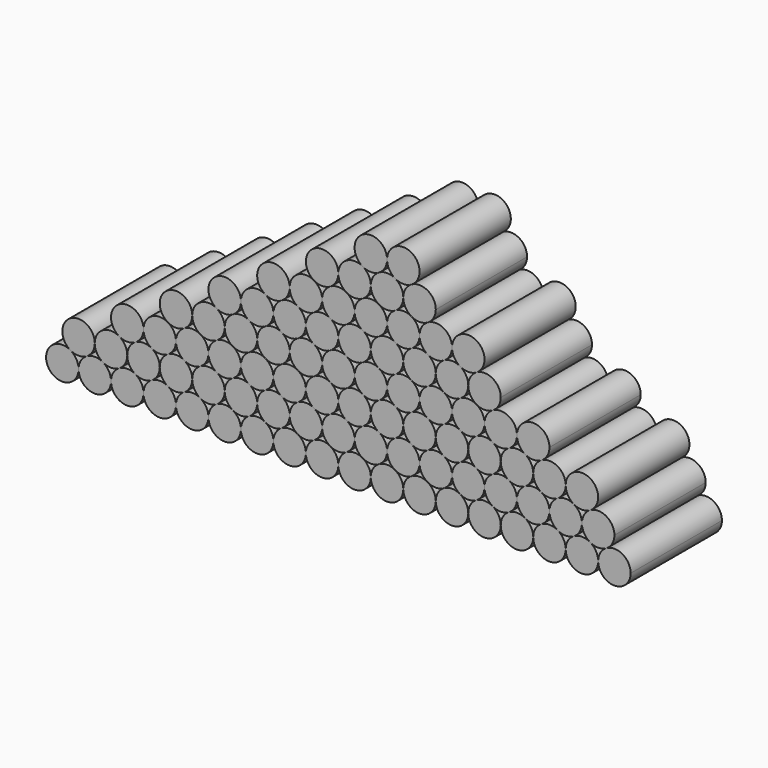
from build123d import *

# Parameters (mm, degrees)
F1_DEPTH = 65


with BuildPart() as f1:
    # F0 (on Front) → F1 (new body)
    with BuildSketch(Plane.XZ):
        with BuildLine():
            ThreePointArc((94.3613596421, 104.9688568004), (90.9756243137, 101.583121778), (89.7363591594, 96.9581215367))
            ThreePointArc((89.7363591594, 96.9581215367), (98.9863591594, 87.7081215367), (108.2363591594, 96.9581215367))
            ThreePointArc((108.2363591594, 96.9581215367), (103.6113594008, 104.9688563823), (94.3613596421, 104.9688568004))
        make_face()
        with BuildLine():
            ThreePointArc((48.1113591587, 137.0117964621), (52.7363591594, 135.7725314467), (57.3613591601, 137.0117964621))
            ThreePointArc((57.3613591601, 137.0117964621), (60.7470941446, 140.397531447), (61.9863591594, 145.0225314467))
            ThreePointArc((61.9863591594, 145.0225314467), (52.7363591594, 154.2725314467), (43.4863591594, 145.0225314467))
            ThreePointArc((43.4863591594, 145.0225314467), (44.7256241742, 140.397531447), (48.1113591587, 137.0117964621))
        make_face()
        with BuildLine():
            ThreePointArc((-25.8886414057, 201.097676668), (-21.2636411008, 199.8584113267), (-16.6386407261, 201.0976764078))
            ThreePointArc((-16.6386407261, 201.0976764078), (-13.2529058226, 204.483411384), (-12.0136408406, 209.1084113267))
            ThreePointArc((-12.0136408406, 209.1084113267), (-21.2636408406, 218.3584113267), (-30.5136408406, 209.1084113267))
            ThreePointArc((-30.5136408406, 209.1084113267), (-29.2743759887, 204.4834116093), (-25.8886414057, 201.097676668))
        make_face()
        with BuildLine():
            ThreePointArc((11.1113595071, 169.054736201), (15.7363595326, 167.8154713867), (20.361359458, 169.0547365741))
            ThreePointArc((20.361359458, 169.0547365741), (23.7470942306, 172.440471536), (24.9863591594, 177.0654713867))
            ThreePointArc((24.9863591594, 177.0654713867), (15.7363591594, 186.3154713867), (6.4863591594, 177.0654713867))
            ThreePointArc((6.4863591594, 177.0654713867), (7.7256242748, 172.4404712129), (11.1113595071, 169.054736201))
        make_face()
        with BuildLine():
            ThreePointArc((-197.0136408406, 112.9795915067), (-210.8886408403, 120.9903264919), (-210.8886408413, 104.9688565221))
            ThreePointArc((-210.8886408413, 104.9688565221), (-206.2636409659, 103.7295915067), (-201.6386410569, 104.9688563968))
            ThreePointArc((-201.6386410569, 104.9688563968), (-198.252905918, 108.3545913985), (-197.0136408406, 112.9795915067))
        make_face()
        with BuildLine():
            ThreePointArc((-183.1386408399, 120.9903264913), (-178.5136408406, 119.7510614767), (-173.8886408413, 120.9903264913))
            ThreePointArc((-173.8886408413, 120.9903264913), (-170.5029058558, 124.3760614763), (-169.2636408406, 129.0010614767))
            ThreePointArc((-169.2636408406, 129.0010614767), (-183.138640841, 137.0117964615), (-183.1386408399, 120.9903264913))
        make_face()
        with BuildLine():
            ThreePointArc((-155.3886408399, 137.0117964613), (-150.7636408406, 135.7725314467), (-146.1386408413, 137.0117964613))
            ThreePointArc((-146.1386408413, 137.0117964613), (-142.7529058558, 140.3975314464), (-141.5136408406, 145.0225314467))
            ThreePointArc((-141.5136408406, 145.0225314467), (-155.388640841, 153.0332664315), (-155.3886408399, 137.0117964613))
        make_face()
        with BuildLine():
            ThreePointArc((-127.6386408399, 153.0332664313), (-123.0136408406, 151.7940014167), (-118.3886408413, 153.0332664313))
            ThreePointArc((-118.3886408413, 153.0332664313), (-115.0029058558, 156.4190014164), (-113.7636408406, 161.0440014167))
            ThreePointArc((-113.7636408406, 161.0440014167), (-127.638640841, 169.0547364015), (-127.6386408399, 153.0332664313))
        make_face()
        with BuildLine():
            ThreePointArc((-86.0136408406, 177.0654713867), (-99.888640841, 185.0762063715), (-99.8886408399, 169.0547364013))
            ThreePointArc((-99.8886408399, 169.0547364013), (-95.2636408406, 167.8154713867), (-90.6386408413, 169.0547364013))
            ThreePointArc((-90.6386408413, 169.0547364013), (-87.2529058558, 172.4404713864), (-86.0136408406, 177.0654713867))
        make_face()
        with BuildLine():
            ThreePointArc((-58.2636408406, 193.0869413567), (-72.1386405587, 201.0976765045), (-72.1386414043, 185.0762066972))
            ThreePointArc((-72.1386414043, 185.0762066972), (-67.5136407818, 183.8369413567), (-62.8886401751, 185.076206756))
            ThreePointArc((-62.8886401751, 185.076206756), (-59.5029056635, 188.4619416895), (-58.2636408406, 193.0869413567))
        make_face()
        with BuildLine():
            ThreePointArc((-44.3886404911, 201.0976761399), (-39.7636403903, 199.8584113267), (-35.1386404101, 201.0976765903))
            ThreePointArc((-35.1386404101, 201.0976765903), (-31.7529057313, 204.483411542), (-30.5136408406, 209.1084113267))
            ThreePointArc((-30.5136408406, 209.1084113267), (-44.3886410154, 217.1191462109), (-44.3886404911, 201.0976761399))
        make_face()
        with BuildLine():
            ThreePointArc((75.8613592919, 120.9903264151), (80.4863592363, 119.7510614767), (85.1113591601, 120.9903264921))
            ThreePointArc((85.1113591601, 120.9903264921), (88.4970941446, 124.376061477), (89.7363591594, 129.0010614767))
            ThreePointArc((89.7363591594, 129.0010614767), (80.4863591594, 138.2510614767), (71.2363591594, 129.0010614767))
            ThreePointArc((71.2363591594, 129.0010614767), (72.4756242127, 124.3760614104), (75.8613592919, 120.9903264151))
        make_face()
        with BuildLine():
            ThreePointArc((71.2363591594, 96.9581215367), (80.4863591594, 87.7081215367), (89.7363591594, 96.9581215367))
            ThreePointArc((89.7363591594, 96.9581215367), (88.4970943958, 101.5831211012), (85.1113600303, 104.9688560188))
            ThreePointArc((85.1113600303, 104.9688560188), (80.4863599409, 106.2081215367), (75.8613596421, 104.9688568004))
            ThreePointArc((75.8613596421, 104.9688568004), (72.4756243137, 101.583121778), (71.2363591594, 96.9581215367))
        make_face()
        with BuildLine():
            ThreePointArc((34.2363591594, 96.9581215367), (43.4863591594, 87.7081215367), (52.7363591594, 96.9581215367))
            ThreePointArc((52.7363591594, 96.9581215367), (51.4970944116, 101.5831210738), (48.1113600851, 104.9688559872))
            ThreePointArc((48.1113600851, 104.9688559872), (43.4863593684, 106.2081215367), (38.8613585957, 104.9688561962))
            ThreePointArc((38.8613585957, 104.9688561962), (35.4756240116, 101.5831212548), (34.2363591594, 96.9581215367))
        make_face()
        with BuildLine():
            ThreePointArc((15.7363591594, 96.9581215367), (24.9863591594, 87.7081215367), (34.2363591594, 96.9581215367))
            ThreePointArc((34.2363591594, 96.9581215367), (32.9970943988, 101.5831210961), (29.6113600405, 104.968856013))
            ThreePointArc((29.6113600405, 104.968856013), (24.9863592931, 106.2081215367), (20.3613585098, 104.9688561466))
            ThreePointArc((20.3613585098, 104.9688561466), (16.9756239869, 101.5831212119), (15.7363591594, 96.9581215367))
        make_face()
        with BuildLine():
            ThreePointArc((52.7363591594, 96.9581215367), (61.9863591594, 87.7081215367), (71.2363591594, 96.9581215367))
            ThreePointArc((71.2363591594, 96.9581215367), (69.9970944022, 101.5831210901), (66.6113600525, 104.968856006))
            ThreePointArc((66.6113600525, 104.968856006), (61.9863592726, 106.2081215367), (57.3613584624, 104.9688561193))
            ThreePointArc((57.3613584624, 104.9688561193), (53.9756239732, 101.5831211882), (52.7363591594, 96.9581215367))
        make_face()
        with BuildLine():
            ThreePointArc((-113.7636408406, 96.9581215367), (-104.5136408406, 87.7081215367), (-95.2636408406, 96.9581215367))
            ThreePointArc((-95.2636408406, 96.9581215367), (-96.5029058558, 101.583121537), (-99.8886408413, 104.9688565221))
            ThreePointArc((-99.8886408413, 104.9688565221), (-104.5136408406, 106.2081215367), (-109.1386408399, 104.9688565221))
            ThreePointArc((-109.1386408399, 104.9688565221), (-112.5243758254, 101.583121537), (-113.7636408406, 96.9581215367))
        make_face()
        with BuildLine():
            ThreePointArc((-95.2636408406, 96.9581215367), (-86.0136408406, 87.7081215367), (-76.7636408406, 96.9581215367))
            ThreePointArc((-76.7636408406, 96.9581215367), (-78.0029058528, 101.5831215319), (-81.388640831, 104.9688565161))
            ThreePointArc((-81.388640831, 104.9688565161), (-86.0136405564, 106.2081215367), (-90.6386403578, 104.9688568004))
            ThreePointArc((-90.6386403578, 104.9688568004), (-94.0243756863, 101.583121778), (-95.2636408406, 96.9581215367))
        make_face()
        with BuildLine():
            ThreePointArc((-76.7636408406, 96.9581215367), (-67.5136408406, 87.7081215367), (-58.2636408406, 96.9581215367))
            ThreePointArc((-58.2636408406, 96.9581215367), (-59.5029057551, 101.5831213626), (-62.8886404925, 104.9688563207))
            ThreePointArc((-62.8886404925, 104.9688563207), (-67.5136406392, 106.2081215367), (-72.1386408399, 104.9688565221))
            ThreePointArc((-72.1386408399, 104.9688565221), (-75.5243758254, 101.583121537), (-76.7636408406, 96.9581215367))
        make_face()
        with BuildLine():
            ThreePointArc((-58.2636408406, 96.9581215367), (-49.0136408406, 87.7081215367), (-39.7636408406, 96.9581215367))
            ThreePointArc((-39.7636408406, 96.9581215367), (-41.0029057637, 101.5831213774), (-44.3886405222, 104.9688563378))
            ThreePointArc((-44.3886405222, 104.9688563378), (-49.0136408578, 106.2081215367), (-53.6386411888, 104.9688563207))
            ThreePointArc((-53.6386411888, 104.9688563207), (-57.0243759261, 101.5831213626), (-58.2636408406, 96.9581215367))
        make_face()
        with BuildLine():
            ThreePointArc((-39.7636408406, 96.9581215367), (-30.5136408406, 87.7081215367), (-21.2636408406, 96.9581215367))
            ThreePointArc((-21.2636408406, 96.9581215367), (-22.5029057222, 101.5831213057), (-25.8886403787, 104.968856255))
            ThreePointArc((-25.8886403787, 104.968856255), (-30.5136403721, 106.2081215367), (-35.1386404911, 104.9688567235))
            ThreePointArc((-35.1386404911, 104.9688567235), (-38.5243757247, 101.5831217114), (-39.7636408406, 96.9581215367))
        make_face()
        with BuildLine():
            ThreePointArc((-21.2636408406, 96.9581215367), (-12.0136408406, 87.7081215367), (-2.7636408406, 96.9581215367))
            ThreePointArc((-2.7636408406, 96.9581215367), (-4.0029056931, 101.5831212551), (-7.3886402775, 104.9688561966))
            ThreePointArc((-7.3886402775, 104.9688561966), (-12.0136406984, 106.2081215367), (-16.6386411573, 104.9688563388))
            ThreePointArc((-16.6386411573, 104.9688563388), (-20.024375917, 101.5831213783), (-21.2636408406, 96.9581215367))
        make_face()
        with BuildLine():
            ThreePointArc((85.1113600303, 104.9688560188), (89.7363599409, 103.7295915067), (94.3613596421, 104.9688568004))
            ThreePointArc((94.3613596421, 104.9688568004), (97.7470942838, 108.3545917481), (98.9863591594, 112.9795915067))
            ThreePointArc((98.9863591594, 112.9795915067), (94.3613591597, 120.9903264915), (85.1113591601, 120.9903264921))
            ThreePointArc((85.1113591601, 120.9903264921), (81.7256241746, 117.604591507), (80.4863591594, 112.9795915067))
            ThreePointArc((80.4863591594, 112.9795915067), (81.7256244258, 108.3545910712), (85.1113600303, 104.9688560188))
        make_face()
        with BuildLine():
            ThreePointArc((-2.7636408406, 96.9581215367), (6.4863591594, 87.7081215367), (15.7363591594, 96.9581215367))
            ThreePointArc((15.7363591594, 96.9581215367), (14.4970942484, 101.5831213566), (11.1113595196, 104.9688563137))
            ThreePointArc((11.1113595196, 104.9688563137), (6.4863591482, 106.2081215367), (1.8613587798, 104.9688563025))
            ThreePointArc((1.8613587798, 104.9688563025), (-1.5243759352, 101.5831213469), (-2.7636408406, 96.9581215367))
        make_face()
        with BuildLine():
            ThreePointArc((-206.2636408406, 96.9581215367), (-197.0136408406, 87.7081215367), (-187.7636408406, 96.9581215367))
            ThreePointArc((-187.7636408406, 96.9581215367), (-189.0029057551, 101.5831213626), (-192.3886404925, 104.9688563207))
            ThreePointArc((-192.3886404925, 104.9688563207), (-197.0136407645, 106.2081215367), (-201.6386410569, 104.9688563968))
            ThreePointArc((-201.6386410569, 104.9688563968), (-205.024375888, 101.5831214285), (-206.2636408406, 96.9581215367))
        make_face()
        with BuildLine():
            ThreePointArc((-187.7636408406, 96.9581215367), (-178.5136408406, 87.7081215367), (-169.2636408406, 96.9581215367))
            ThreePointArc((-169.2636408406, 96.9581215367), (-170.5029058554, 101.5831215363), (-173.8886408399, 104.9688565213))
            ThreePointArc((-173.8886408399, 104.9688565213), (-178.5136408398, 106.2081215367), (-183.1386408399, 104.9688565221))
            ThreePointArc((-183.1386408399, 104.9688565221), (-186.5243758254, 101.583121537), (-187.7636408406, 96.9581215367))
        make_face()
        with BuildLine():
            ThreePointArc((-169.2636408406, 96.9581215367), (-160.0136408406, 87.7081215367), (-150.7636408406, 96.9581215367))
            ThreePointArc((-150.7636408406, 96.9581215367), (-152.0029058472, 101.5831215222), (-155.3886408116, 104.9688565049))
            ThreePointArc((-155.3886408116, 104.9688565049), (-160.0136406229, 106.2081215367), (-164.6386404925, 104.9688567227))
            ThreePointArc((-164.6386404925, 104.9688567227), (-168.0243757251, 101.5831217107), (-169.2636408406, 96.9581215367))
        make_face()
        with BuildLine():
            ThreePointArc((-150.7636408406, 96.9581215367), (-141.5136408406, 87.7081215367), (-132.2636408406, 96.9581215367))
            ThreePointArc((-132.2636408406, 96.9581215367), (-133.5029057936, 101.5831214292), (-136.8886406257, 104.9688563976))
            ThreePointArc((-136.8886406257, 104.9688563976), (-141.5136407161, 106.2081215367), (-146.1386408399, 104.9688565221))
            ThreePointArc((-146.1386408399, 104.9688565221), (-149.5243758254, 101.583121537), (-150.7636408406, 96.9581215367))
        make_face()
        with BuildLine():
            ThreePointArc((-132.2636408406, 96.9581215367), (-123.0136408406, 87.7081215367), (-113.7636408406, 96.9581215367))
            ThreePointArc((-113.7636408406, 96.9581215367), (-115.0029058558, 101.583121537), (-118.3886408413, 104.9688565221))
            ThreePointArc((-118.3886408413, 104.9688565221), (-123.0136405576, 106.2081215367), (-127.6386403497, 104.9688568051))
            ThreePointArc((-127.6386403497, 104.9688568051), (-131.0243756839, 101.5831217821), (-132.2636408406, 96.9581215367))
        make_face()
        with BuildLine():
            ThreePointArc((20.3613591587, 153.0332664321), (24.9863592839, 151.7940014167), (29.6113593757, 153.0332665566))
            ThreePointArc((29.6113593757, 153.0332665566), (32.9970942068, 156.4190015248), (34.2363591594, 161.0440014167))
            ThreePointArc((34.2363591594, 161.0440014167), (29.6113593087, 169.0547363155), (20.361359458, 169.0547365741))
            ThreePointArc((20.361359458, 169.0547365741), (16.9756242606, 165.669001566), (15.7363591594, 161.0440014167))
            ThreePointArc((15.7363591594, 161.0440014167), (16.9756241742, 156.4190014171), (20.3613591587, 153.0332664321))
        make_face()
        with BuildLine():
            ThreePointArc((-16.6386408413, 185.0762063721), (-12.0136407594, 183.8369413567), (-7.3886406993, 185.0762064533))
            ThreePointArc((-7.3886406993, 185.0762064533), (-4.0029058148, 188.4619414274), (-2.7636408406, 193.0869413567))
            ThreePointArc((-2.7636408406, 193.0869413567), (-7.3886407834, 201.0976763087), (-16.6386407261, 201.0976764078))
            ThreePointArc((-16.6386407261, 201.0976764078), (-20.0243757926, 197.711941414), (-21.2636408406, 193.0869413567))
            ThreePointArc((-21.2636408406, 193.0869413567), (-20.0243758258, 188.4619413571), (-16.6386408413, 185.0762063721))
        make_face()
        with BuildLine():
            ThreePointArc((-197.0136408406, 112.9795915067), (-195.7743757251, 108.3545913326), (-192.3886404925, 104.9688563207))
            ThreePointArc((-192.3886404925, 104.9688563207), (-187.7636406392, 103.7295915067), (-183.1386408399, 104.9688565221))
            ThreePointArc((-183.1386408399, 104.9688565221), (-179.7529058554, 108.354591507), (-178.5136408406, 112.9795915067))
            ThreePointArc((-178.5136408406, 112.9795915067), (-179.7529058554, 117.6045915063), (-183.1386408399, 120.9903264913))
            ThreePointArc((-183.1386408399, 120.9903264913), (-192.3886408403, 120.9903264919), (-197.0136408406, 112.9795915067))
        make_face()
        with BuildLine():
            ThreePointArc((-169.2636408406, 129.0010614767), (-168.0243757636, 124.3760613692), (-164.6386406257, 120.9903263676))
            ThreePointArc((-164.6386406257, 120.9903263676), (-160.0136407161, 119.7510614767), (-155.3886408399, 120.9903264921))
            ThreePointArc((-155.3886408399, 120.9903264921), (-152.0029058554, 124.376061477), (-150.7636408406, 129.0010614767))
            ThreePointArc((-150.7636408406, 129.0010614767), (-152.0029058554, 133.6260614763), (-155.3886408399, 137.0117964613))
            ThreePointArc((-155.3886408399, 137.0117964613), (-164.6386408403, 137.0117964619), (-169.2636408406, 129.0010614767))
        make_face()
        with BuildLine():
            ThreePointArc((57.3613591273, 120.9903265102), (61.9863591888, 119.7510614767), (66.6113592424, 120.9903265396))
            ThreePointArc((66.6113592424, 120.9903265396), (69.9970941684, 124.3760615182), (71.2363591594, 129.0010614767))
            ThreePointArc((71.2363591594, 129.0010614767), (66.6113591597, 137.0117964615), (57.3613591601, 137.0117964621))
            ThreePointArc((57.3613591601, 137.0117964621), (53.9756241746, 133.626061477), (52.7363591594, 129.0010614767))
            ThreePointArc((52.7363591594, 129.0010614767), (53.9756241651, 124.3760614928), (57.3613591273, 120.9903265102))
        make_face()
        with BuildLine():
            ThreePointArc((-141.5136408406, 145.0225314467), (-140.2743757251, 140.3975312726), (-136.8886404925, 137.0117962607))
            ThreePointArc((-136.8886404925, 137.0117962607), (-132.2636406392, 135.7725314467), (-127.6386408399, 137.0117964621))
            ThreePointArc((-127.6386408399, 137.0117964621), (-124.2529058554, 140.397531447), (-123.0136408406, 145.0225314467))
            ThreePointArc((-123.0136408406, 145.0225314467), (-124.2529058554, 149.6475314464), (-127.6386408399, 153.0332664313))
            ThreePointArc((-127.6386408399, 153.0332664313), (-136.8886408403, 153.0332664319), (-141.5136408406, 145.0225314467))
        make_face()
        with BuildLine():
            ThreePointArc((-109.138640708, 153.0332663552), (-104.5136407637, 151.7940014167), (-99.8886408399, 153.0332664321))
            ThreePointArc((-99.8886408399, 153.0332664321), (-96.5029058554, 156.4190014171), (-95.2636408406, 161.0440014167))
            ThreePointArc((-95.2636408406, 161.0440014167), (-96.5029058554, 165.6690014164), (-99.8886408399, 169.0547364013))
            ThreePointArc((-99.8886408399, 169.0547364013), (-109.1386408403, 169.0547364019), (-113.7636408406, 161.0440014167))
            ThreePointArc((-113.7636408406, 161.0440014167), (-112.5243757873, 156.4190013504), (-109.138640708, 153.0332663552))
        make_face()
        with BuildLine():
            ThreePointArc((29.6113595134, 137.0117962573), (34.2363593679, 135.7725314467), (38.8613591664, 137.0117964657))
            ThreePointArc((38.8613591664, 137.0117964657), (42.2470941464, 140.3975314502), (43.4863591594, 145.0225314467))
            ThreePointArc((43.4863591594, 145.0225314467), (38.8613592675, 153.0332663693), (29.6113593757, 153.0332665566))
            ThreePointArc((29.6113593757, 153.0332665566), (26.2256242368, 149.6475315548), (24.9863591594, 145.0225314467))
            ThreePointArc((24.9863591594, 145.0225314467), (26.2256242766, 140.3975312697), (29.6113595134, 137.0117962573))
        make_face()
        with BuildLine():
            ThreePointArc((-86.0136408406, 177.0654713867), (-84.7743757873, 172.4404713203), (-81.3886407078, 169.0547363251))
            ThreePointArc((-81.3886407078, 169.0547363251), (-76.7636407636, 167.8154713867), (-72.1386408399, 169.0547364021))
            ThreePointArc((-72.1386408399, 169.0547364021), (-68.7529058554, 172.4404713871), (-67.5136408406, 177.0654713867))
            ThreePointArc((-67.5136408406, 177.0654713867), (-68.7529060183, 181.6904716686), (-72.1386414043, 185.0762066972))
            ThreePointArc((-72.1386414043, 185.0762066972), (-81.3886411225, 185.076206209), (-86.0136408406, 177.0654713867))
        make_face()
        with BuildLine():
            ThreePointArc((-12.0136408406, 177.0654713867), (-10.7743759018, 172.4404715188), (-7.3886411047, 169.0547365542))
            ThreePointArc((-7.3886411047, 169.0547365542), (-2.7636411967, 167.8154713867), (1.8613588067, 169.0547361981))
            ThreePointArc((1.8613588067, 169.0547361981), (5.2470940426, 172.4404712104), (6.4863591594, 177.0654713867))
            ThreePointArc((6.4863591594, 177.0654713867), (1.8613592301, 185.0762063309), (-7.3886406993, 185.0762064533))
            ThreePointArc((-7.3886406993, 185.0762064533), (-10.7743757848, 181.6904714574), (-12.0136408406, 177.0654713867))
        make_face()
        with BuildLine():
            ThreePointArc((-53.6386408155, 185.0762063572), (-49.0136407012, 183.8369413567), (-44.3886406243, 185.0762064966))
            ThreePointArc((-44.3886406243, 185.0762064966), (-41.0029057932, 188.4619414649), (-39.7636408406, 193.0869413567))
            ThreePointArc((-39.7636408406, 193.0869413567), (-41.0029057547, 197.711941182), (-44.3886404911, 201.0976761399))
            ThreePointArc((-44.3886404911, 201.0976761399), (-53.6386406659, 201.0976764426), (-58.2636408406, 193.0869413567))
            ThreePointArc((-58.2636408406, 193.0869413567), (-57.0243758184, 188.4619413442), (-53.6386408155, 185.0762063572))
        make_face()
        with BuildLine():
            ThreePointArc((-86.0136408406, 145.0225314467), (-84.7743758258, 140.397531447), (-81.3886408413, 137.0117964621))
            ThreePointArc((-81.3886408413, 137.0117964621), (-76.7636408406, 135.7725314467), (-72.1386408399, 137.0117964621))
            ThreePointArc((-72.1386408399, 137.0117964621), (-68.7529058554, 140.397531447), (-67.5136408406, 145.0225314467))
            ThreePointArc((-67.5136408406, 145.0225314467), (-68.7529058558, 149.647531447), (-72.1386408413, 153.0332664321))
            ThreePointArc((-72.1386408413, 153.0332664321), (-76.7636407161, 154.2725314467), (-81.3886406243, 153.0332665566))
            ThreePointArc((-81.3886406243, 153.0332665566), (-84.7743757632, 149.6475315548), (-86.0136408406, 145.0225314467))
        make_face()
        with BuildLine():
            ThreePointArc((15.7363591594, 129.0010614767), (16.9756241742, 124.376061477), (20.3613591587, 120.9903264921))
            ThreePointArc((20.3613591587, 120.9903264921), (24.9863592069, 119.7510614767), (29.6113592424, 120.9903265396))
            ThreePointArc((29.6113592424, 120.9903265396), (32.9970941684, 124.3760615182), (34.2363591594, 129.0010614767))
            ThreePointArc((34.2363591594, 129.0010614767), (32.9970942466, 133.6260612997), (29.6113595134, 137.0117962573))
            ThreePointArc((29.6113595134, 137.0117962573), (24.9863592389, 138.2510614767), (20.3613589431, 137.0117963368))
            ThreePointArc((20.3613589431, 137.0117963368), (16.975624112, 133.6260613685), (15.7363591594, 129.0010614767))
        make_face()
        with BuildLine():
            ThreePointArc((29.6113600405, 104.968856013), (34.2363593426, 103.7295915067), (38.8613585957, 104.9688561962))
            ThreePointArc((38.8613585957, 104.9688561962), (42.2470939817, 108.3545912248), (43.4863591594, 112.9795915067))
            ThreePointArc((43.4863591594, 112.9795915067), (42.2470941827, 117.6045914404), (38.8613592919, 120.9903264151))
            ThreePointArc((38.8613592919, 120.9903264151), (34.2363592839, 122.2295915067), (29.6113592424, 120.9903265396))
            ThreePointArc((29.6113592424, 120.9903265396), (26.2256241984, 117.6045915482), (24.9863591594, 112.9795915067))
            ThreePointArc((24.9863591594, 112.9795915067), (26.2256244287, 108.3545910661), (29.6113600405, 104.968856013))
        make_face()
        with BuildLine():
            ThreePointArc((-12.0136408406, 112.9795915067), (-10.7743756631, 108.3545912251), (-7.3886402775, 104.9688561966))
            ThreePointArc((-7.3886402775, 104.9688561966), (-2.7636407347, 103.7295915067), (1.8613587798, 104.9688563025))
            ThreePointArc((1.8613587798, 104.9688563025), (5.2470940348, 108.3545913169), (6.4863591594, 112.9795915067))
            ThreePointArc((6.4863591594, 112.9795915067), (5.2470941451, 117.6045915055), (1.8613591618, 120.9903264903))
            ThreePointArc((1.8613591618, 120.9903264903), (-2.7636408396, 122.2295915067), (-7.3886408413, 120.9903264913))
            ThreePointArc((-7.3886408413, 120.9903264913), (-10.7743758258, 117.6045915063), (-12.0136408406, 112.9795915067))
        make_face()
        with BuildLine():
            ThreePointArc((-21.2636408406, 129.0010614767), (-20.0243758254, 124.3760614763), (-16.6386408399, 120.9903264913))
            ThreePointArc((-16.6386408399, 120.9903264913), (-12.0136408406, 119.7510614767), (-7.3886408413, 120.9903264913))
            ThreePointArc((-7.3886408413, 120.9903264913), (-4.0029058558, 124.3760614763), (-2.7636408406, 129.0010614767))
            ThreePointArc((-2.7636408406, 129.0010614767), (-4.0029057941, 133.6260613701), (-7.3886406275, 137.0117963386))
            ThreePointArc((-7.3886406275, 137.0117963386), (-12.0136407171, 138.2510614767), (-16.6386408399, 137.0117964621))
            ThreePointArc((-16.6386408399, 137.0117964621), (-20.0243758254, 133.626061477), (-21.2636408406, 129.0010614767))
        make_face()
        with BuildLine():
            ThreePointArc((43.4863591594, 112.9795915067), (44.7256244416, 108.3545910438), (48.1113600851, 104.9688559872))
            ThreePointArc((48.1113600851, 104.9688559872), (52.7363592914, 103.7295915067), (57.3613584624, 104.9688561193))
            ThreePointArc((57.3613584624, 104.9688561193), (60.7470939432, 108.3545911582), (61.9863591594, 112.9795915067))
            ThreePointArc((61.9863591594, 112.9795915067), (60.7470941351, 117.6045915227), (57.3613591273, 120.9903265102))
            ThreePointArc((57.3613591273, 120.9903265102), (52.7363591412, 122.2295915067), (48.1113591601, 120.9903264921))
            ThreePointArc((48.1113591601, 120.9903264921), (44.7256241746, 117.604591507), (43.4863591594, 112.9795915067))
        make_face()
        with BuildLine():
            ThreePointArc((-7.3886406275, 137.0117963386), (-2.7636406402, 135.7725314467), (1.8613592934, 137.0117965391))
            ThreePointArc((1.8613592934, 137.0117965391), (5.2470941831, 140.3975315137), (6.4863591594, 145.0225314467))
            ThreePointArc((6.4863591594, 145.0225314467), (5.2470941442, 149.647531447), (1.8613591587, 153.0332664321))
            ThreePointArc((1.8613591587, 153.0332664321), (-2.7636407594, 154.2725314467), (-7.3886406993, 153.0332665133))
            ThreePointArc((-7.3886406993, 153.0332665133), (-10.7743757848, 149.6475315174), (-12.0136408406, 145.0225314467))
            ThreePointArc((-12.0136408406, 145.0225314467), (-10.7743757641, 140.3975313401), (-7.3886406275, 137.0117963386))
        make_face()
        with BuildLine():
            ThreePointArc((-49.0136408406, 177.0654713867), (-47.7743758184, 172.4404713742), (-44.3886408155, 169.0547363872))
            ThreePointArc((-44.3886408155, 169.0547363872), (-39.7636407488, 167.8154713867), (-35.1386407067, 169.054736479))
            ThreePointArc((-35.1386407067, 169.054736479), (-31.7529058169, 172.4404714537), (-30.5136408406, 177.0654713867))
            ThreePointArc((-30.5136408406, 177.0654713867), (-31.752905918, 181.6904714949), (-35.1386410569, 185.0762064966))
            ThreePointArc((-35.1386410569, 185.0762064966), (-39.7636408406, 186.3154713867), (-44.3886406243, 185.0762064966))
            ThreePointArc((-44.3886406243, 185.0762064966), (-47.7743757632, 181.6904714949), (-49.0136408406, 177.0654713867))
        make_face()
        with BuildLine():
            ThreePointArc((-132.2636408406, 129.0010614767), (-131.0243758258, 124.376061477), (-127.6386408413, 120.9903264921))
            ThreePointArc((-127.6386408413, 120.9903264921), (-123.0136408406, 119.7510614767), (-118.3886408399, 120.9903264921))
            ThreePointArc((-118.3886408399, 120.9903264921), (-115.0029058554, 124.376061477), (-113.7636408406, 129.0010614767))
            ThreePointArc((-113.7636408406, 129.0010614767), (-115.0029057936, 133.6260613692), (-118.3886406257, 137.0117963376))
            ThreePointArc((-118.3886406257, 137.0117963376), (-123.0136407161, 138.2510614767), (-127.6386408399, 137.0117964621))
            ThreePointArc((-127.6386408399, 137.0117964621), (-131.0243758254, 133.626061477), (-132.2636408406, 129.0010614767))
        make_face()
        with BuildLine():
            ThreePointArc((-21.2636408406, 161.0440014167), (-20.0243758258, 156.4190014171), (-16.6386408413, 153.0332664321))
            ThreePointArc((-16.6386408413, 153.0332664321), (-12.0136407594, 151.7940014167), (-7.3886406993, 153.0332665133))
            ThreePointArc((-7.3886406993, 153.0332665133), (-4.0029058148, 156.4190014874), (-2.7636408406, 161.0440014167))
            ThreePointArc((-2.7636408406, 161.0440014167), (-4.0029059318, 165.6690015487), (-7.3886411047, 169.0547365542))
            ThreePointArc((-7.3886411047, 169.0547365542), (-12.0136408682, 170.2940014167), (-16.6386406243, 169.0547365266))
            ThreePointArc((-16.6386406243, 169.0547365266), (-20.0243757632, 165.6690015248), (-21.2636408406, 161.0440014167))
        make_face()
        with BuildLine():
            ThreePointArc((-86.0136408406, 112.9795915067), (-84.7743758229, 108.3545915019), (-81.388640831, 104.9688565161))
            ThreePointArc((-81.388640831, 104.9688565161), (-76.7636408347, 103.7295915067), (-72.1386408399, 104.9688565221))
            ThreePointArc((-72.1386408399, 104.9688565221), (-68.7529058554, 108.354591507), (-67.5136408406, 112.9795915067))
            ThreePointArc((-67.5136408406, 112.9795915067), (-68.7529060187, 117.6045917892), (-72.1386414057, 120.9903268179))
            ThreePointArc((-72.1386414057, 120.9903268179), (-76.7636409175, 122.2295915067), (-81.3886404087, 120.990326741))
            ThreePointArc((-81.3886404087, 120.990326741), (-84.7743757009, 117.6045917226), (-86.0136408406, 112.9795915067))
        make_face()
        with BuildLine():
            ThreePointArc((-76.7636408406, 129.0010614767), (-75.5243759887, 124.3760617592), (-72.1386414057, 120.9903268179))
            ThreePointArc((-72.1386414057, 120.9903268179), (-67.513641156, 119.7510614767), (-62.8886408219, 120.9903265025))
            ThreePointArc((-62.8886408219, 120.9903265025), (-59.5029058502, 124.3760614861), (-58.2636408406, 129.0010614767))
            ThreePointArc((-58.2636408406, 129.0010614767), (-59.502905918, 133.6260615848), (-62.8886410569, 137.0117965866))
            ThreePointArc((-62.8886410569, 137.0117965866), (-67.5136409651, 138.2510614767), (-72.1386408399, 137.0117964621))
            ThreePointArc((-72.1386408399, 137.0117964621), (-75.5243758254, 133.626061477), (-76.7636408406, 129.0010614767))
        make_face()
        with BuildLine():
            ThreePointArc((-35.1386410569, 185.0762064966), (-30.5136408994, 183.8369413567), (-25.8886407261, 185.0762064378))
            ThreePointArc((-25.8886407261, 185.0762064378), (-22.5029058226, 188.461941414), (-21.2636408406, 193.0869413567))
            ThreePointArc((-21.2636408406, 193.0869413567), (-22.5029060187, 197.7119416393), (-25.8886414057, 201.097676668))
            ThreePointArc((-25.8886414057, 201.097676668), (-30.5136409183, 202.3369413567), (-35.1386404101, 201.0976765903))
            ThreePointArc((-35.1386404101, 201.0976765903), (-38.5243757013, 197.711941572), (-39.7636408406, 193.0869413567))
            ThreePointArc((-39.7636408406, 193.0869413567), (-38.524375888, 188.4619414649), (-35.1386410569, 185.0762064966))
        make_face()
        with BuildLine():
            ThreePointArc((-95.2636408406, 161.0440014167), (-94.0243758202, 156.4190014073), (-90.6386408219, 153.0332664209))
            ThreePointArc((-90.6386408219, 153.0332664209), (-86.0136407049, 151.7940014167), (-81.3886406243, 153.0332665566))
            ThreePointArc((-81.3886406243, 153.0332665566), (-78.0029057932, 156.4190015248), (-76.7636408406, 161.0440014167))
            ThreePointArc((-76.7636408406, 161.0440014167), (-78.0029058173, 165.6690013503), (-81.3886407078, 169.0547363251))
            ThreePointArc((-81.3886407078, 169.0547363251), (-86.0136407643, 170.2940014167), (-90.6386408413, 169.0547364013))
            ThreePointArc((-90.6386408413, 169.0547364013), (-94.0243758258, 165.6690014164), (-95.2636408406, 161.0440014167))
        make_face()
        with BuildLine():
            ThreePointArc((34.2363591594, 129.0010614767), (35.4756242127, 124.3760614104), (38.8613592919, 120.9903264151))
            ThreePointArc((38.8613592919, 120.9903264151), (43.4863592363, 119.7510614767), (48.1113591601, 120.9903264921))
            ThreePointArc((48.1113591601, 120.9903264921), (51.4970941446, 124.376061477), (52.7363591594, 129.0010614767))
            ThreePointArc((52.7363591594, 129.0010614767), (51.4970941442, 133.626061477), (48.1113591587, 137.0117964621))
            ThreePointArc((48.1113591587, 137.0117964621), (43.4863591631, 138.2510614767), (38.8613591664, 137.0117964657))
            ThreePointArc((38.8613591664, 137.0117964657), (35.4756241764, 133.6260614802), (34.2363591594, 129.0010614767))
        make_face()
        with BuildLine():
            ThreePointArc((6.4863591594, 145.0225314467), (7.7256241742, 140.397531447), (11.1113591587, 137.0117964621))
            ThreePointArc((11.1113591587, 137.0117964621), (15.7363590341, 135.7725314467), (20.3613589431, 137.0117963368))
            ThreePointArc((20.3613589431, 137.0117963368), (23.747094082, 140.3975313386), (24.9863591594, 145.0225314467))
            ThreePointArc((24.9863591594, 145.0225314467), (23.7470941442, 149.647531447), (20.3613591587, 153.0332664321))
            ThreePointArc((20.3613591587, 153.0332664321), (15.7363592076, 154.2725314467), (11.1113592435, 153.0332664803))
            ThreePointArc((11.1113592435, 153.0332664803), (7.7256241987, 149.6475314888), (6.4863591594, 145.0225314467))
        make_face()
        with BuildLine():
            ThreePointArc((-104.5136408406, 145.0225314467), (-103.2743759265, 140.3975316215), (-99.8886411901, 137.0117966635))
            ThreePointArc((-99.8886411901, 137.0117966635), (-95.2636407637, 135.7725314467), (-90.6386403579, 137.0117967404))
            ThreePointArc((-90.6386403579, 137.0117967404), (-87.2529057162, 140.3975316881), (-86.0136408406, 145.0225314467))
            ThreePointArc((-86.0136408406, 145.0225314467), (-87.2529058502, 149.6475314373), (-90.6386408219, 153.0332664209))
            ThreePointArc((-90.6386408219, 153.0332664209), (-95.2636408294, 154.2725314467), (-99.8886408399, 153.0332664321))
            ThreePointArc((-99.8886408399, 153.0332664321), (-103.2743758254, 149.647531447), (-104.5136408406, 145.0225314467))
        make_face()
        with BuildLine():
            ThreePointArc((-49.0136408406, 112.9795915067), (-47.7743757337, 108.3545913474), (-44.3886405222, 104.9688563378))
            ThreePointArc((-44.3886405222, 104.9688563378), (-39.763640455, 103.7295915067), (-35.1386404911, 104.9688567235))
            ThreePointArc((-35.1386404911, 104.9688567235), (-31.7529057547, 108.3545916814), (-30.5136408406, 112.9795915067))
            ThreePointArc((-30.5136408406, 112.9795915067), (-31.7529058554, 117.6045915063), (-35.1386408399, 120.9903264913))
            ThreePointArc((-35.1386408399, 120.9903264913), (-39.7636408398, 122.2295915067), (-44.3886408399, 120.9903264921))
            ThreePointArc((-44.3886408399, 120.9903264921), (-47.7743758254, 117.604591507), (-49.0136408406, 112.9795915067))
        make_face()
        with BuildLine():
            ThreePointArc((11.1113595196, 104.9688563137), (15.7363589923, 103.7295915067), (20.3613585098, 104.9688561466))
            ThreePointArc((20.3613585098, 104.9688561466), (23.7470939569, 108.3545911819), (24.9863591594, 112.9795915067))
            ThreePointArc((24.9863591594, 112.9795915067), (23.7470941442, 117.604591507), (20.3613591587, 120.9903264921))
            ThreePointArc((20.3613591587, 120.9903264921), (15.736359158, 122.2295915067), (11.1113591576, 120.9903264907))
            ThreePointArc((11.1113591576, 120.9903264907), (7.7256241739, 117.6045915058), (6.4863591594, 112.9795915067))
            ThreePointArc((6.4863591594, 112.9795915067), (7.7256242784, 108.3545913266), (11.1113595196, 104.9688563137))
        make_face()
        with BuildLine():
            ThreePointArc((-67.5136408406, 145.0225314467), (-66.274375888, 140.3975315548), (-62.8886410569, 137.0117965866))
            ThreePointArc((-62.8886410569, 137.0117965866), (-58.2636410412, 135.7725314467), (-53.6386409718, 137.0117963859))
            ThreePointArc((-53.6386409718, 137.0117963859), (-50.2529058935, 140.3975313811), (-49.0136408406, 145.0225314467))
            ThreePointArc((-49.0136408406, 145.0225314467), (-50.2529057936, 149.6475313392), (-53.6386406257, 153.0332663076))
            ThreePointArc((-53.6386406257, 153.0332663076), (-58.263640668, 154.2725314467), (-62.8886407565, 153.0332664803))
            ThreePointArc((-62.8886407565, 153.0332664803), (-66.2743758013, 149.6475314888), (-67.5136408406, 145.0225314467))
        make_face()
        with BuildLine():
            ThreePointArc((-150.7636408406, 129.0010614767), (-149.5243757873, 124.3760614104), (-146.1386407081, 120.9903264151))
            ThreePointArc((-146.1386407081, 120.9903264151), (-141.5136407376, 119.7510614767), (-136.8886407947, 120.9903265182))
            ThreePointArc((-136.8886407947, 120.9903265182), (-133.5029058424, 124.3760614996), (-132.2636408406, 129.0010614767))
            ThreePointArc((-132.2636408406, 129.0010614767), (-133.5029057551, 133.6260613026), (-136.8886404925, 137.0117962607))
            ThreePointArc((-136.8886404925, 137.0117962607), (-141.51364064, 138.2510614767), (-146.1386408413, 137.0117964613))
            ThreePointArc((-146.1386408413, 137.0117964613), (-149.5243758258, 133.6260614763), (-150.7636408406, 129.0010614767))
        make_face()
        with BuildLine():
            ThreePointArc((-118.3886408413, 104.9688565221), (-113.7636408406, 103.7295915067), (-109.1386408399, 104.9688565221))
            ThreePointArc((-109.1386408399, 104.9688565221), (-105.7529058554, 108.354591507), (-104.5136408406, 112.9795915067))
            ThreePointArc((-104.5136408406, 112.9795915067), (-105.7529059565, 117.6045916814), (-109.1386411901, 120.9903266935))
            ThreePointArc((-109.1386411901, 120.9903266935), (-113.763641042, 122.2295915067), (-118.3886408399, 120.9903264921))
            ThreePointArc((-118.3886408399, 120.9903264921), (-121.7743758254, 117.604591507), (-123.0136408406, 112.9795915067))
            ThreePointArc((-123.0136408406, 112.9795915067), (-121.7743758258, 108.354591507), (-118.3886408413, 104.9688565221))
        make_face()
        with BuildLine():
            ThreePointArc((-104.5136408406, 112.9795915067), (-103.2743758258, 108.354591507), (-99.8886408413, 104.9688565221))
            ThreePointArc((-99.8886408413, 104.9688565221), (-95.2636405623, 103.7295915067), (-90.6386403578, 104.9688568004))
            ThreePointArc((-90.6386403578, 104.9688568004), (-87.2529057162, 108.3545917481), (-86.0136408406, 112.9795915067))
            ThreePointArc((-86.0136408406, 112.9795915067), (-87.2529058558, 117.604591507), (-90.6386408413, 120.9903264921))
            ThreePointArc((-90.6386408413, 120.9903264921), (-95.2636408406, 122.2295915067), (-99.8886408399, 120.9903264921))
            ThreePointArc((-99.8886408399, 120.9903264921), (-103.2743758254, 117.604591507), (-104.5136408406, 112.9795915067))
        make_face()
        with BuildLine():
            ThreePointArc((-141.5136408406, 112.9795915067), (-140.2743757636, 108.3545913992), (-136.8886406257, 104.9688563976))
            ThreePointArc((-136.8886406257, 104.9688563976), (-132.2636404331, 103.7295915067), (-127.6386403497, 104.9688568051))
            ThreePointArc((-127.6386403497, 104.9688568051), (-124.2529057139, 108.3545917521), (-123.0136408406, 112.9795915067))
            ThreePointArc((-123.0136408406, 112.9795915067), (-124.2529058558, 117.604591507), (-127.6386408413, 120.9903264921))
            ThreePointArc((-127.6386408413, 120.9903264921), (-132.2636408145, 122.2295915067), (-136.8886407947, 120.9903265182))
            ThreePointArc((-136.8886407947, 120.9903265182), (-140.2743758124, 117.6045915296), (-141.5136408406, 112.9795915067))
        make_face()
        with BuildLine():
            ThreePointArc((-2.7636408406, 161.0440014167), (-1.5243758258, 156.4190014171), (1.8613591587, 153.0332664321))
            ThreePointArc((1.8613591587, 153.0332664321), (6.4863592076, 151.7940014167), (11.1113592435, 153.0332664803))
            ThreePointArc((11.1113592435, 153.0332664803), (14.4970941687, 156.4190014588), (15.7363591594, 161.0440014167))
            ThreePointArc((15.7363591594, 161.0440014167), (14.4970942448, 165.6690012428), (11.1113595071, 169.054736201))
            ThreePointArc((11.1113595071, 169.054736201), (6.4863591565, 170.2940014167), (1.8613588067, 169.0547361981))
            ThreePointArc((1.8613588067, 169.0547361981), (-1.5243759274, 165.6690012403), (-2.7636408406, 161.0440014167))
        make_face()
        with BuildLine():
            ThreePointArc((-113.7636408406, 129.0010614767), (-112.5243759265, 124.3760616514), (-109.1386411901, 120.9903266935))
            ThreePointArc((-109.1386411901, 120.9903266935), (-104.513641042, 119.7510614767), (-99.8886408399, 120.9903264921))
            ThreePointArc((-99.8886408399, 120.9903264921), (-96.5029058554, 124.376061477), (-95.2636408406, 129.0010614767))
            ThreePointArc((-95.2636408406, 129.0010614767), (-96.5029059565, 133.6260616514), (-99.8886411901, 137.0117966635))
            ThreePointArc((-99.8886411901, 137.0117966635), (-104.5136409175, 138.2510614767), (-109.1386406243, 137.0117965866))
            ThreePointArc((-109.1386406243, 137.0117965866), (-112.5243757632, 133.6260615848), (-113.7636408406, 129.0010614767))
        make_face()
        with BuildLine():
            ThreePointArc((-39.7636408406, 129.0010614767), (-38.5243758254, 124.3760614763), (-35.1386408399, 120.9903264913))
            ThreePointArc((-35.1386408399, 120.9903264913), (-30.5136408528, 119.7510614767), (-25.8886408625, 120.9903264791))
            ThreePointArc((-25.8886408625, 120.9903264791), (-22.5029058619, 124.3760614657), (-21.2636408406, 129.0010614767))
            ThreePointArc((-21.2636408406, 129.0010614767), (-22.5029057551, 133.6260613026), (-25.8886404925, 137.0117962607))
            ThreePointArc((-25.8886404925, 137.0117962607), (-30.5136408406, 138.2510614767), (-35.1386411888, 137.0117962607))
            ThreePointArc((-35.1386411888, 137.0117962607), (-38.5243759261, 133.6260613026), (-39.7636408406, 129.0010614767))
        make_face()
        with BuildLine():
            ThreePointArc((-58.2636408406, 161.0440014167), (-57.0243757636, 156.4190013093), (-53.6386406257, 153.0332663076))
            ThreePointArc((-53.6386406257, 153.0332663076), (-49.0136407161, 151.7940014167), (-44.3886408399, 153.0332664321))
            ThreePointArc((-44.3886408399, 153.0332664321), (-41.0029058554, 156.4190014171), (-39.7636408406, 161.0440014167))
            ThreePointArc((-39.7636408406, 161.0440014167), (-41.0029058483, 165.6690014041), (-44.3886408155, 169.0547363872))
            ThreePointArc((-44.3886408155, 169.0547363872), (-49.0136407012, 170.2940014167), (-53.6386406243, 169.0547365266))
            ThreePointArc((-53.6386406243, 169.0547365266), (-57.0243757632, 165.6690015248), (-58.2636408406, 161.0440014167))
        make_face()
        with BuildLine():
            ThreePointArc((-39.7636408406, 161.0440014167), (-38.524375888, 156.4190015248), (-35.1386410569, 153.0332665566))
            ThreePointArc((-35.1386410569, 153.0332665566), (-30.5136409651, 151.7940014167), (-25.8886408399, 153.0332664321))
            ThreePointArc((-25.8886408399, 153.0332664321), (-22.5029058554, 156.4190014171), (-21.2636408406, 161.0440014167))
            ThreePointArc((-21.2636408406, 161.0440014167), (-22.5029057551, 165.6690012426), (-25.8886404925, 169.0547362007))
            ThreePointArc((-25.8886404925, 169.0547362007), (-30.5136405623, 170.2940014167), (-35.1386407067, 169.054736479))
            ThreePointArc((-35.1386407067, 169.054736479), (-38.524375787, 165.6690014837), (-39.7636408406, 161.0440014167))
        make_face()
        with BuildLine():
            ThreePointArc((-30.5136408406, 177.0654713867), (-29.2743757251, 172.4404712126), (-25.8886404925, 169.0547362007))
            ThreePointArc((-25.8886404925, 169.0547362007), (-21.2636405147, 167.8154713867), (-16.6386406243, 169.0547365266))
            ThreePointArc((-16.6386406243, 169.0547365266), (-13.2529057932, 172.4404714949), (-12.0136408406, 177.0654713867))
            ThreePointArc((-12.0136408406, 177.0654713867), (-13.2529058558, 181.6904713871), (-16.6386408413, 185.0762063721))
            ThreePointArc((-16.6386408413, 185.0762063721), (-21.2636407749, 186.3154713867), (-25.8886407261, 185.0762064378))
            ThreePointArc((-25.8886407261, 185.0762064378), (-29.2743757926, 181.690471444), (-30.5136408406, 177.0654713867))
        make_face()
        with BuildLine():
            ThreePointArc((-160.0136408406, 112.9795915067), (-158.7743758172, 108.3545914922), (-155.3886408116, 104.9688565049))
            ThreePointArc((-155.3886408116, 104.9688565049), (-150.7636408235, 103.7295915067), (-146.1386408399, 104.9688565221))
            ThreePointArc((-146.1386408399, 104.9688565221), (-142.7529058554, 108.354591507), (-141.5136408406, 112.9795915067))
            ThreePointArc((-141.5136408406, 112.9795915067), (-142.7529058173, 117.6045914404), (-146.1386407081, 120.9903264151))
            ThreePointArc((-146.1386407081, 120.9903264151), (-150.7636407637, 122.2295915067), (-155.3886408399, 120.9903264921))
            ThreePointArc((-155.3886408399, 120.9903264921), (-158.7743758254, 117.604591507), (-160.0136408406, 112.9795915067))
        make_face()
        with BuildLine():
            ThreePointArc((-44.3886404879, 137.011796258), (-39.763640838, 135.7725314467), (-35.1386411888, 137.0117962607))
            ThreePointArc((-35.1386411888, 137.0117962607), (-31.7529059561, 140.3975312726), (-30.5136408406, 145.0225314467))
            ThreePointArc((-30.5136408406, 145.0225314467), (-31.752905918, 149.6475315548), (-35.1386410569, 153.0332665566))
            ThreePointArc((-35.1386410569, 153.0332665566), (-39.7636409651, 154.2725314467), (-44.3886408399, 153.0332664321))
            ThreePointArc((-44.3886408399, 153.0332664321), (-47.7743758254, 149.647531447), (-49.0136408406, 145.0225314467))
            ThreePointArc((-49.0136408406, 145.0225314467), (-47.7743757238, 140.3975312703), (-44.3886404879, 137.011796258))
        make_face()
        with BuildLine():
            ThreePointArc((66.6113600525, 104.968856006), (71.2363599538, 103.7295915067), (75.8613596421, 104.9688568004))
            ThreePointArc((75.8613596421, 104.9688568004), (79.2470942838, 108.3545917481), (80.4863591594, 112.9795915067))
            ThreePointArc((80.4863591594, 112.9795915067), (79.2470941827, 117.6045914404), (75.8613592919, 120.9903264151))
            ThreePointArc((75.8613592919, 120.9903264151), (71.2363592839, 122.2295915067), (66.6113592424, 120.9903265396))
            ThreePointArc((66.6113592424, 120.9903265396), (63.2256241984, 117.6045915482), (61.9863591594, 112.9795915067))
            ThreePointArc((61.9863591594, 112.9795915067), (63.2256244322, 108.3545910601), (66.6113600525, 104.968856006))
        make_face()
        with BuildLine():
            ThreePointArc((-30.5136408406, 112.9795915067), (-29.2743756923, 108.3545912757), (-25.8886403787, 104.968856255))
            ThreePointArc((-25.8886403787, 104.968856255), (-21.2636407567, 103.7295915067), (-16.6386411573, 104.9688563388))
            ThreePointArc((-16.6386411573, 104.9688563388), (-13.252905947, 108.3545913483), (-12.0136408406, 112.9795915067))
            ThreePointArc((-12.0136408406, 112.9795915067), (-13.2529058554, 117.6045915063), (-16.6386408399, 120.9903264913))
            ThreePointArc((-16.6386408399, 120.9903264913), (-21.2636408528, 122.2295915067), (-25.8886408625, 120.9903264791))
            ThreePointArc((-25.8886408625, 120.9903264791), (-29.2743758319, 117.6045914957), (-30.5136408406, 112.9795915067))
        make_face()
        with BuildLine():
            ThreePointArc((-67.5136408406, 112.9795915067), (-66.2743757251, 108.3545913326), (-62.8886404925, 104.9688563207))
            ThreePointArc((-62.8886404925, 104.9688563207), (-58.2636408406, 103.7295915067), (-53.6386411888, 104.9688563207))
            ThreePointArc((-53.6386411888, 104.9688563207), (-50.2529059561, 108.3545913326), (-49.0136408406, 112.9795915067))
            ThreePointArc((-49.0136408406, 112.9795915067), (-50.2529058554, 117.6045915063), (-53.6386408399, 120.9903264913))
            ThreePointArc((-53.6386408399, 120.9903264913), (-58.2636408294, 122.2295915067), (-62.8886408219, 120.9903265025))
            ThreePointArc((-62.8886408219, 120.9903265025), (-66.2743758202, 117.6045915161), (-67.5136408406, 112.9795915067))
        make_face()
        with BuildLine():
            ThreePointArc((-67.5136408406, 177.0654713867), (-66.274375758, 172.4404712695), (-62.8886406063, 169.0547362664))
            ThreePointArc((-62.8886406063, 169.0547362664), (-58.2636405804, 167.8154713867), (-53.6386406243, 169.0547365266))
            ThreePointArc((-53.6386406243, 169.0547365266), (-50.2529057932, 172.4404714949), (-49.0136408406, 177.0654713867))
            ThreePointArc((-49.0136408406, 177.0654713867), (-50.2529058483, 181.6904713742), (-53.6386408155, 185.0762063572))
            ThreePointArc((-53.6386408155, 185.0762063572), (-58.2636404419, 186.3154713867), (-62.8886401751, 185.076206756))
            ThreePointArc((-62.8886401751, 185.076206756), (-66.2743756335, 181.6904717195), (-67.5136408406, 177.0654713867))
        make_face()
        with BuildLine():
            ThreePointArc((-76.7636408406, 161.0440014167), (-75.5243758258, 156.4190014171), (-72.1386408413, 153.0332664321))
            ThreePointArc((-72.1386408413, 153.0332664321), (-67.5136407924, 151.7940014167), (-62.8886407565, 153.0332664803))
            ThreePointArc((-62.8886407565, 153.0332664803), (-59.5029058313, 156.4190014588), (-58.2636408406, 161.0440014167))
            ThreePointArc((-58.2636408406, 161.0440014167), (-59.502905788, 165.6690012995), (-62.8886406063, 169.0547362664))
            ThreePointArc((-62.8886406063, 169.0547362664), (-67.5136407049, 170.2940014167), (-72.1386408399, 169.0547364021))
            ThreePointArc((-72.1386408399, 169.0547364021), (-75.5243758254, 165.6690014171), (-76.7636408406, 161.0440014167))
        make_face()
        with BuildLine():
            ThreePointArc((-178.5136408406, 112.9795915067), (-177.2743758254, 108.3545915063), (-173.8886408399, 104.9688565213))
            ThreePointArc((-173.8886408399, 104.9688565213), (-169.2636406392, 103.7295915067), (-164.6386404925, 104.9688567227))
            ThreePointArc((-164.6386404925, 104.9688567227), (-161.2529057551, 108.3545916807), (-160.0136408406, 112.9795915067))
            ThreePointArc((-160.0136408406, 112.9795915067), (-161.2529057936, 117.6045913992), (-164.6386406257, 120.9903263676))
            ThreePointArc((-164.6386406257, 120.9903263676), (-169.2636407169, 122.2295915067), (-173.8886408413, 120.9903264913))
            ThreePointArc((-173.8886408413, 120.9903264913), (-177.2743758258, 117.6045915063), (-178.5136408406, 112.9795915067))
        make_face()
        with BuildLine():
            ThreePointArc((-123.0136408406, 145.0225314467), (-121.7743757636, 140.3975313392), (-118.3886406257, 137.0117963376))
            ThreePointArc((-118.3886406257, 137.0117963376), (-113.7636405917, 135.7725314467), (-109.1386406243, 137.0117965866))
            ThreePointArc((-109.1386406243, 137.0117965866), (-105.7529057932, 140.3975315548), (-104.5136408406, 145.0225314467))
            ThreePointArc((-104.5136408406, 145.0225314467), (-105.7529058173, 149.6475313804), (-109.138640708, 153.0332663552))
            ThreePointArc((-109.138640708, 153.0332663552), (-113.7636407645, 154.2725314467), (-118.3886408413, 153.0332664313))
            ThreePointArc((-118.3886408413, 153.0332664313), (-121.7743758258, 149.6475314464), (-123.0136408406, 145.0225314467))
        make_face()
        with BuildLine():
            ThreePointArc((-90.6386408413, 120.9903264921), (-86.0136405917, 119.7510614767), (-81.3886404087, 120.990326741))
            ThreePointArc((-81.3886404087, 120.990326741), (-78.0029057309, 124.3760616926), (-76.7636408406, 129.0010614767))
            ThreePointArc((-76.7636408406, 129.0010614767), (-78.0029058558, 133.626061477), (-81.3886408413, 137.0117964621))
            ThreePointArc((-81.3886408413, 137.0117964621), (-86.0136405623, 138.2510614767), (-90.6386403579, 137.0117967404))
            ThreePointArc((-90.6386403579, 137.0117967404), (-94.0243756863, 133.6260617181), (-95.2636408406, 129.0010614767))
            ThreePointArc((-95.2636408406, 129.0010614767), (-94.0243758258, 124.376061477), (-90.6386408413, 120.9903264921))
        make_face()
        with BuildLine():
            ThreePointArc((-25.8886404925, 137.0117962607), (-21.2636406392, 135.7725314467), (-16.6386408399, 137.0117964621))
            ThreePointArc((-16.6386408399, 137.0117964621), (-13.2529058554, 140.397531447), (-12.0136408406, 145.0225314467))
            ThreePointArc((-12.0136408406, 145.0225314467), (-13.2529058558, 149.647531447), (-16.6386408413, 153.0332664321))
            ThreePointArc((-16.6386408413, 153.0332664321), (-21.2636408406, 154.2725314467), (-25.8886408399, 153.0332664321))
            ThreePointArc((-25.8886408399, 153.0332664321), (-29.2743758254, 149.647531447), (-30.5136408406, 145.0225314467))
            ThreePointArc((-30.5136408406, 145.0225314467), (-29.2743757251, 140.3975312726), (-25.8886404925, 137.0117962607))
        make_face()
        with BuildLine():
            ThreePointArc((-53.6386408399, 120.9903264913), (-49.0136408398, 119.7510614767), (-44.3886408399, 120.9903264921))
            ThreePointArc((-44.3886408399, 120.9903264921), (-41.0029058554, 124.376061477), (-39.7636408406, 129.0010614767))
            ThreePointArc((-39.7636408406, 129.0010614767), (-41.0029057538, 133.6260613003), (-44.3886404879, 137.011796258))
            ThreePointArc((-44.3886404879, 137.011796258), (-49.0136407127, 138.2510614767), (-53.6386409718, 137.0117963859))
            ThreePointArc((-53.6386409718, 137.0117963859), (-57.0243758635, 133.6260614111), (-58.2636408406, 129.0010614767))
            ThreePointArc((-58.2636408406, 129.0010614767), (-57.0243758254, 124.3760614763), (-53.6386408399, 120.9903264913))
        make_face()
        with BuildLine():
            ThreePointArc((-2.7636408406, 129.0010614767), (-1.5243758249, 124.3760614755), (1.8613591618, 120.9903264903))
            ThreePointArc((1.8613591618, 120.9903264903), (6.4863591598, 119.7510614767), (11.1113591576, 120.9903264907))
            ThreePointArc((11.1113591576, 120.9903264907), (14.4970941439, 124.3760614758), (15.7363591594, 129.0010614767))
            ThreePointArc((15.7363591594, 129.0010614767), (14.4970941442, 133.626061477), (11.1113591587, 137.0117964621))
            ThreePointArc((11.1113591587, 137.0117964621), (6.4863592364, 138.2510614767), (1.8613592934, 137.0117965391))
            ThreePointArc((1.8613592934, 137.0117965391), (-1.5243757869, 133.6260615437), (-2.7636408406, 129.0010614767))
        make_face()
        with BuildLine():
            ThreePointArc((-210.8886408413, 104.9688565221), (-223.5243758254, 92.3331215363), (-206.2636408406, 96.9581215367))
            ThreePointArc((-206.2636408406, 96.9581215367), (-207.5029058558, 101.583121537), (-210.8886408413, 104.9688565221))
        make_face()
    extrude(amount=F1_DEPTH)


solid = f1.part
